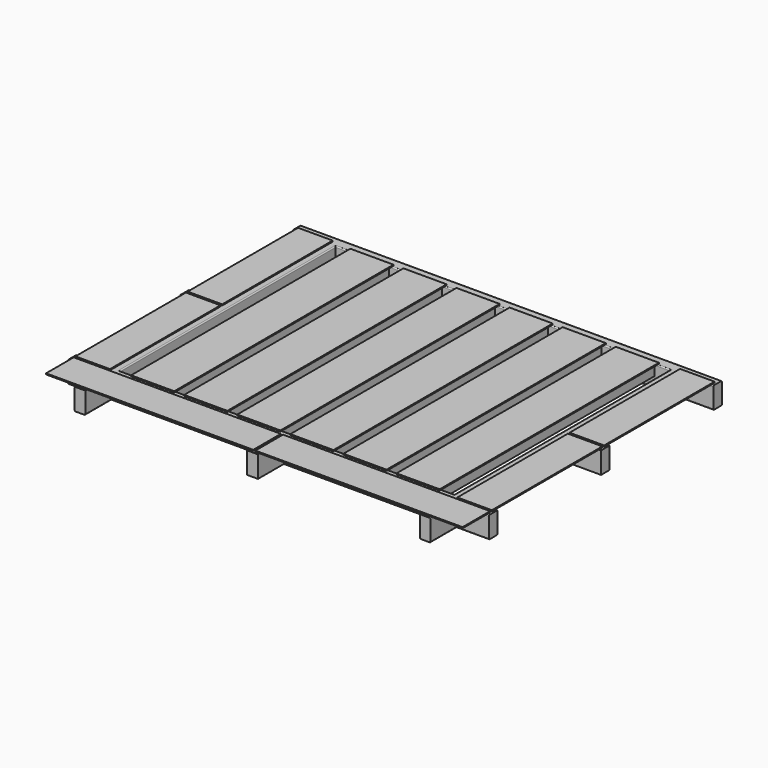
from build123d import *

# Parameters (mm, degrees)
F1_DEPTH = 100
F2_R     = 5
F0_W     = 50
F0_H     = 1250
F3_DEPTH = 50
F5_W     = 960
F5_H     = 160
F5_W_2   = 160
F5_H_2   = 640
F6_DEPTH = 5
F7_W     = 200
F7_H     = 1270
F8_DEPTH = 5


# Not quite as in the source:
# - two fillets or chamfers of one size are made in one step


with BuildPart() as f1:
    # F0 (on Top) → F1 (new body)
    with BuildSketch(Plane.XY):
        Polygon((0, 50), (0, 0), (150, 0), (150, -150), (200, -150), (200, 0), (950, 0), (950, -150), (1000, -150), (1000, 0), (1750, 0), (1750, -150), (1800, -150), (1800, 0), (1950, 0), (1950, 50), (1800, 50), (1800, 650), (1800, 700), (1800, 1300), (1950, 1300), (1950, 1350), (0, 1350), (0, 1300), (150, 1300), (150, 700), (0, 700), (0, 675), (0, 650), (150, 650), (150, 50), align=None)
        Polygon((200, 50), (200, 1300), (273.1, 1300), (323.1, 1300), (396.2, 1300), (446.2, 1300), (519.3, 1300), (569.3, 1300), (642.4, 1300), (692.4, 1300), (765.5, 1300), (815.5, 1300), (888.6, 1300), (938.6, 1300), (1011.7, 1300), (1061.7, 1300), (1134.8, 1300), (1184.8, 1300), (1257.9, 1300), (1307.9, 1300), (1381, 1300), (1431, 1300), (1504.1, 1300), (1554.1, 1300), (1627.2, 1300), (1677.2, 1300), (1750, 1300), (1750, 50), (1677.2, 50), (1627.2, 50), (1554.1, 50), (1504.1, 50), (1431, 50), (1381, 50), (1307.9, 50), (1257.9, 50), (1184.8, 50), (1134.8, 50), (1061.7, 50), (1011.7, 50), (938.6, 50), (888.6, 50), (815.5, 50), (765.5, 50), (692.4, 50), (642.4, 50), (569.3, 50), (519.3, 50), (446.2, 50), (396.2, 50), (323.1, 50), (273.1, 50), align=None, mode=Mode.SUBTRACT)
        Polygon((1950, 700), (1800, 700), (1800, 650), (1950, 650), (1950, 675), align=None)
    extrude(amount=-F1_DEPTH)

    # F2
    f2_edges = [f1.edges().sort_by_distance(p)[0] for p in [
        (75, 1300, 0),
        (975, 1350, 0),
        (975, 1300, 0),
        (200, 675, 0),
        (150, 1000, 0),
        (575, 0, 0),
        (975, 50, 0),
        (75, 50, 0),
        (75, 0, 0),
        (150, -75, 0),
        (1750, 675, 0),
        (1800, 350, 0),
        (1800, 1000, 0),
        (1875, 50, 0),
        (1875, 0, 0),
        (1800, -75, 0),
        (1750, -75, 0),
        (1875, 1300, 0),
        (75, 0, -100),
        (150, -75, -100),
        (200, -75, -100),
        (575, 0, -100),
        (1750, -75, -100),
        (1800, -75, -100),
        (1875, 0, -100),
        (1875, 50, -100),
        (1800, 350, -100),
        (1800, 1000, -100),
        (1875, 1300, -100),
        (975, 1350, -100),
        (75, 1300, -100),
        (150, 1000, -100),
        (75, 50, -100),
        (200, 675, -100),
        (975, 1300, -100),
        (1750, 675, -100),
        (975, 50, -100),
    ]]
    fillet(f2_edges, radius=F2_R)

    # F5 (on Top) → F6 (join)
    with BuildSketch(Plane.XY):
        with Locations((1460, -60)):
            Rectangle(F5_W, F5_H)
        with Locations((490, -60)):
            Rectangle(F5_W, F5_H)
        with Locations((90, 1000)):
            Rectangle(F5_W_2, F5_H_2)
        with Locations((90, 350)):
            Rectangle(F5_W_2, F5_H_2)
        with Locations((1860, 350)):
            Rectangle(F5_W_2, F5_H_2)
        with Locations((1860, 1000)):
            Rectangle(F5_W_2, F5_H_2)
    extrude(amount=F6_DEPTH)


with BuildPart() as f3:
    # F0 (on Top) → F3 (new body)
    with BuildSketch(Plane.XY):
        with Locations((298.1, 675)):
            Rectangle(F0_W, F0_H)
    extrude(amount=-F3_DEPTH)


with BuildPart() as f3b:
    # F0 (on Top) → F3, piece 2 (new body)
    with BuildSketch(Plane.XY):
        with Locations((421.2, 675)):
            Rectangle(F0_W, F0_H)
    extrude(amount=-F3_DEPTH)


with BuildPart() as f3c:
    # F0 (on Top) → F3, piece 3 (new body)
    with BuildSketch(Plane.XY):
        with Locations((544.3, 675)):
            Rectangle(F0_W, F0_H)
    extrude(amount=-F3_DEPTH)


with BuildPart() as f3d:
    # F0 (on Top) → F3, piece 4 (new body)
    with BuildSketch(Plane.XY):
        with Locations((667.4, 675)):
            Rectangle(F0_W, F0_H)
    extrude(amount=-F3_DEPTH)


with BuildPart() as f3e:
    # F0 (on Top) → F3, piece 5 (new body)
    with BuildSketch(Plane.XY):
        with Locations((790.5, 675)):
            Rectangle(F0_W, F0_H)
    extrude(amount=-F3_DEPTH)


with BuildPart() as f3f:
    # F0 (on Top) → F3, piece 6 (new body)
    with BuildSketch(Plane.XY):
        with Locations((913.6, 675)):
            Rectangle(F0_W, F0_H)
    extrude(amount=-F3_DEPTH)


with BuildPart() as f3g:
    # F0 (on Top) → F3, piece 7 (new body)
    with BuildSketch(Plane.XY):
        with Locations((1036.7, 675)):
            Rectangle(F0_W, F0_H)
    extrude(amount=-F3_DEPTH)


with BuildPart() as f3h:
    # F0 (on Top) → F3, piece 8 (new body)
    with BuildSketch(Plane.XY):
        with Locations((1159.8, 675)):
            Rectangle(F0_W, F0_H)
    extrude(amount=-F3_DEPTH)


with BuildPart() as f3i:
    # F0 (on Top) → F3, piece 9 (new body)
    with BuildSketch(Plane.XY):
        with Locations((1282.9, 675)):
            Rectangle(F0_W, F0_H)
    extrude(amount=-F3_DEPTH)


with BuildPart() as f3j:
    # F0 (on Top) → F3, piece 10 (new body)
    with BuildSketch(Plane.XY):
        with Locations((1406, 675)):
            Rectangle(F0_W, F0_H)
    extrude(amount=-F3_DEPTH)


with BuildPart() as f3k:
    # F0 (on Top) → F3, piece 11 (new body)
    with BuildSketch(Plane.XY):
        with Locations((1529.1, 675)):
            Rectangle(F0_W, F0_H)
    extrude(amount=-F3_DEPTH)


with BuildPart() as f3l:
    # F0 (on Top) → F3, piece 12 (new body)
    with BuildSketch(Plane.XY):
        with Locations((1652.2, 675)):
            Rectangle(F0_W, F0_H)
    extrude(amount=-F3_DEPTH)


with BuildPart() as f8:
    # F7 (on Top) → F8 (new body)
    with BuildSketch(Plane.XY):
        with Locations((360, 675)):
            Rectangle(F7_W, F7_H)
    extrude(amount=F8_DEPTH)


with BuildPart() as f8b:
    # F7 (on Top) → F8, piece 2 (new body)
    with BuildSketch(Plane.XY):
        with Locations((606, 675)):
            Rectangle(F7_W, F7_H)
    extrude(amount=F8_DEPTH)


with BuildPart() as f8c:
    # F7 (on Top) → F8, piece 3 (new body)
    with BuildSketch(Plane.XY):
        with Locations((852, 675)):
            Rectangle(F7_W, F7_H)
    extrude(amount=F8_DEPTH)


with BuildPart() as f8d:
    # F7 (on Top) → F8, piece 4 (new body)
    with BuildSketch(Plane.XY):
        with Locations((1098, 675)):
            Rectangle(F7_W, F7_H)
    extrude(amount=F8_DEPTH)


with BuildPart() as f8e:
    # F7 (on Top) → F8, piece 5 (new body)
    with BuildSketch(Plane.XY):
        with Locations((1344, 675)):
            Rectangle(F7_W, F7_H)
    extrude(amount=F8_DEPTH)


with BuildPart() as f8f:
    # F7 (on Top) → F8, piece 6 (new body)
    with BuildSketch(Plane.XY):
        with Locations((1590, 675)):
            Rectangle(F7_W, F7_H)
    extrude(amount=F8_DEPTH)


solid = Compound([f1.part, f3.part, f3b.part, f3c.part, f3d.part, f3e.part, f3f.part, f3g.part, f3h.part, f3i.part, f3j.part, f3k.part, f3l.part, f8.part, f8b.part, f8c.part, f8d.part, f8e.part, f8f.part])
